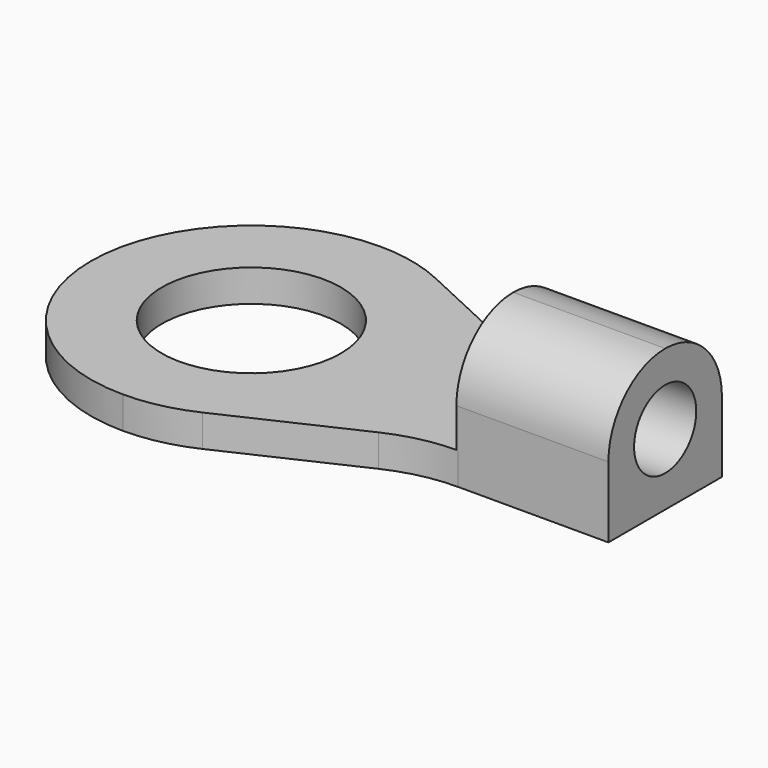
from build123d import *

# Parameters (mm, degrees)
F0_R     = 2.65
F1_DEPTH = 0.95
F3_DEPTH = 3.25
F4_R     = 2.09999
F5_R     = 1.15
F6_DEPTH = 25


# Not quite as in the source:
# - a fillet or chamfer is up to 0.001 mm smaller than in the source, because OpenCascade refuses the exact size


with BuildPart() as f1:
    # F0 (on Top) → F1 (new body)
    with BuildSketch(Plane.XY):
        with BuildLine():
            Line((12.5502312096, 2.65), (17, 2.65))
            Line((17, 2.65), (17, 6.85))
            Line((17, 6.85), (12.5502312096, 6.85))
            ThreePointArc((12.5502312096, 6.85), (11.5247662629, 6.9620131907), (10.5476657796, 7.2927698345))
            Line((10.5476657796, 7.2927698345), (6.75256543, 9.0572301655))
            ThreePointArc((6.75256543, 9.0572301655), (5.7754649467, 9.3879868093), (4.75, 9.5))
            ThreePointArc((4.75, 9.5), (1.3912427894, 8.1087572106), (0, 4.75))
            ThreePointArc((0, 4.75), (1.3912427894, 1.3912427894), (4.75, 0))
            ThreePointArc((4.75, 0), (5.7754649467, 0.1120131907), (6.75256543, 0.4427698345))
            Line((6.75256543, 0.4427698345), (10.5476657796, 2.2072301655))
            ThreePointArc((10.5476657796, 2.2072301655), (11.5247662629, 2.5379868093), (12.5502312096, 2.65))
        make_face()
        with Locations((4.75, 4.75)):
            Circle(F0_R, mode=Mode.SUBTRACT)
    extrude(amount=F1_DEPTH)

    # F2 (on face) → F3 (join)
    with BuildSketch(Plane.XY.offset(0.95)):
        Polygon((17, 2.65), (17, 6.85), (12.5502312096, 6.85), (12.5, 6.85), (12.5, 2.65), (12.5502312096, 2.65), align=None)
    extrude(amount=F3_DEPTH)

    # F4 (radius 2.1 in the source; OpenCascade refuses exactly that, so slightly less here)
    f4_edges = [f1.edges().sort_by_distance(p)[0] for p in [
        (14.75, 6.85, 4.2),
        (14.75, 2.65, 4.2),
    ]]
    fillet(f4_edges, radius=F4_R)

    # F5 (on face) → F6 (cut)
    with BuildSketch(Plane.YZ.offset(17)):
        with Locations((4.75, 2.1)):
            Circle(F5_R)
    extrude(amount=-F6_DEPTH, mode=Mode.SUBTRACT)


solid = f1.part
